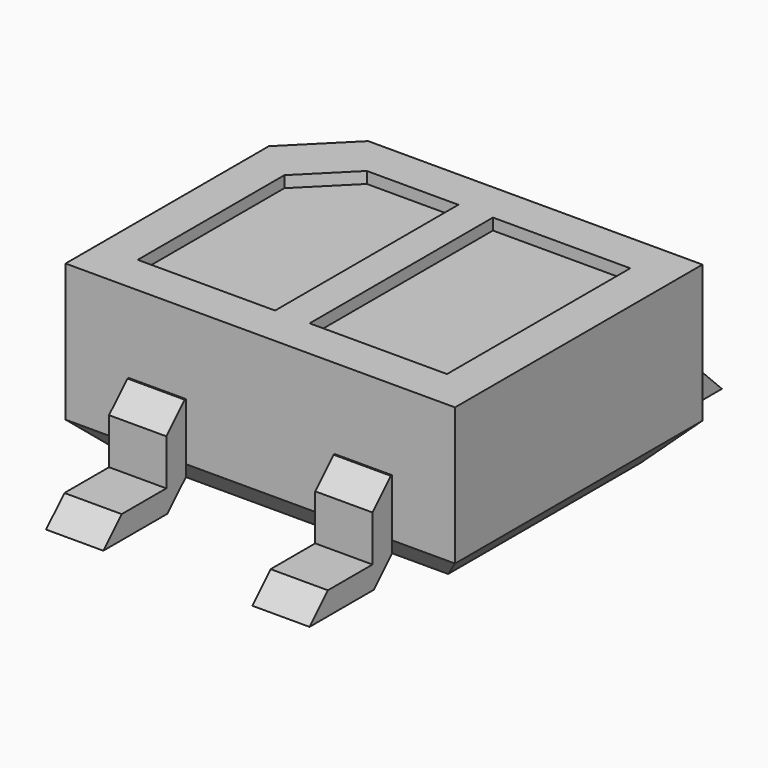
from build123d import *

# Parameters (mm, degrees)
F0_W      = 1.1990487342
F0_H      = 2
F1_DEPTH  = 1.5
F2_DEPTH  = 1.4
F3_SIZE   = 0.3
F0_W_2    = 0.5
F0_H_2    = 0.6870733146
F0_H_3    = 0.2129266854
F4_DEPTH  = 0.2
F5_DEPTH  = 0.8
F6_SIZE   = 0.19999
F6_2_SIZE = 0.19999
F6_3_SIZE = 0.19999
F6_4_SIZE = 0.19999


# Not quite as in the source:
# - a fillet or chamfer is up to 0.001 mm smaller than in the source, because OpenCascade refuses the exact size


with BuildPart() as f1:
    # F0 (on Top) → F1 (new body)
    with BuildSketch(Plane.XY):
        Polygon((1.7, -1.35), (1.7, 1.35), (1.15, 1.35), (0.65, 1.35), (-0.65, 1.35), (-1.15, 1.35), (-1.2177615426, 1.35), (-1.7, 0.8677615426), (-1.7, -1.35), (-1.15, -1.35), (-0.65, -1.35), (0.65, -1.35), (1.15, -1.35), align=None)
        Polygon((-1.35, -1), (-1.35, 0.6), (-0.95, 1), (-0.1509512658, 1), (-0.1509512658, -1), align=None, mode=Mode.SUBTRACT)
        with Locations((0.7504756329, 0)):
            Rectangle(F0_W, F0_H, mode=Mode.SUBTRACT)
    extrude(amount=F1_DEPTH)

    # F0 (on Top) → F2 (join)
    with BuildSketch(Plane.XY):
        Polygon((-0.95, 1), (-1.35, 0.6), (-1.35, -1), (-0.1509512658, -1), (-0.1509512658, 1), align=None)
        with Locations((0.7504756329, 0)):
            Rectangle(F0_W, F0_H)
    extrude(amount=F2_DEPTH)

    # F3
    f3_edges = [f1.edges().sort_by_distance(p)[0] for p in [
        (-1.7, -0.241119, 0),
        (-1.458881, 1.108881, 0),
        (0.241119, 1.35, 0),
        (0, -1.35, 0),
        (1.7, 0, 0),
    ]]
    chamfer(f3_edges, length=F3_SIZE)


with BuildPart() as f4:
    # F0 (on Top) → F4 (new body)
    with BuildSketch(Plane.XY):
        with Locations((-0.9, 1.9064633427)):
            Rectangle(F0_W_2, F0_H_2)
        with Locations((-0.9, 1.4564633427)):
            Rectangle(F0_W_2, F0_H_3)
    extrude(amount=F4_DEPTH)

    # F0 (on Top) → F5, piece 2 (join)
    with BuildSketch(Plane.XY):
        with Locations((-0.9, 1.4564633427)):
            Rectangle(F0_W_2, F0_H_3)
    extrude(amount=F5_DEPTH)

    # F6 (size 0.2 in the source; OpenCascade refuses exactly that, so slightly less here)
    f6_edges = [f4.edges().sort_by_distance(p)[0] for p in [
        (-0.9, 2.25, 0.2),
        (-0.9, 1.35, 0),
        (-0.9, 1.562927, 0.8),
    ]]
    chamfer(f6_edges, length=F6_SIZE)


with BuildPart() as f4b:
    # F0 (on Top) → F4, piece 2 (new body)
    with BuildSketch(Plane.XY):
        with Locations((0.9, 1.9064633427)):
            Rectangle(F0_W_2, F0_H_2)
    extrude(amount=F4_DEPTH)

    # F0 (on Top) → F5 (join)
    with BuildSketch(Plane.XY):
        with Locations((0.9, 1.4564633427)):
            Rectangle(F0_W_2, F0_H_3)
    extrude(amount=F5_DEPTH)

    # F6#2 (size 0.2 in the source; OpenCascade refuses exactly that, so slightly less here)
    f6_2_edges = [f4b.edges().sort_by_distance(p)[0] for p in [
        (0.9, 1.35, 0),
        (0.9, 2.25, 0.2),
        (0.9, 1.562927, 0.8),
    ]]
    chamfer(f6_2_edges, length=F6_2_SIZE)


with BuildPart() as f4c:
    # F0 (on Top) → F4, piece 3 (new body)
    with BuildSketch(Plane.XY):
        with Locations((-0.9, -1.9064633427)):
            Rectangle(F0_W_2, F0_H_2)
        with Locations((-0.9, -1.4564633427)):
            Rectangle(F0_W_2, F0_H_3)
    extrude(amount=F4_DEPTH)

    # F0 (on Top) → F5, piece 3 (join)
    with BuildSketch(Plane.XY):
        with Locations((-0.9, -1.4564633427)):
            Rectangle(F0_W_2, F0_H_3)
    extrude(amount=F5_DEPTH)

    # F6#3 (size 0.2 in the source; OpenCascade refuses exactly that, so slightly less here)
    f6_3_edges = [f4c.edges().sort_by_distance(p)[0] for p in [
        (-0.9, -2.25, 0.2),
        (-0.9, -1.35, 0),
        (-0.9, -1.562927, 0.8),
    ]]
    chamfer(f6_3_edges, length=F6_3_SIZE)


with BuildPart() as f4d:
    # F0 (on Top) → F4, piece 4 (new body)
    with BuildSketch(Plane.XY):
        with Locations((0.9, -1.9064633427)):
            Rectangle(F0_W_2, F0_H_2)
        with Locations((0.9, -1.4564633427)):
            Rectangle(F0_W_2, F0_H_3)
    extrude(amount=F4_DEPTH)

    # F0 (on Top) → F5, piece 4 (join)
    with BuildSketch(Plane.XY):
        with Locations((0.9, -1.4564633427)):
            Rectangle(F0_W_2, F0_H_3)
    extrude(amount=F5_DEPTH)

    # F6#4 (size 0.2 in the source; OpenCascade refuses exactly that, so slightly less here)
    f6_4_edges = [f4d.edges().sort_by_distance(p)[0] for p in [
        (0.9, -2.25, 0.2),
        (0.9, -1.35, 0),
        (0.9, -1.562927, 0.8),
    ]]
    chamfer(f6_4_edges, length=F6_4_SIZE)


solid = Compound([f1.part, f4.part, f4b.part, f4c.part, f4d.part])
